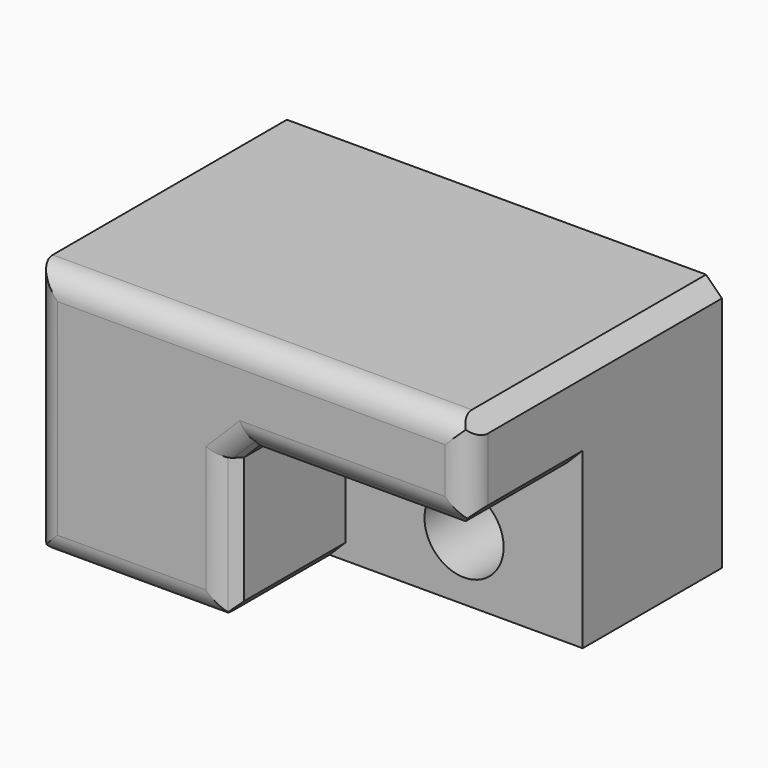
from build123d import *

# Parameters (mm, degrees)
F0_W         = 55
F0_H         = 32
F1_DEPTH     = 40
F2_W         = 30
F2_H         = 18
F3_DEPTH     = 20
F4_R         = 5
F5_DEPTH     = 22.001
F6_SIZE      = 2
F7_T1_DEPTH  = 36
F7_T3_DEPTH  = 45
F7_T5_DEPTH  = 68
F7_T7_DEPTH  = 23
F7_T12_DEPTH = 34.2132034356
F7_T17_DEPTH = 24.2132034356
F7_T22_DEPTH = 13.4214256026
F7_T29_DEPTH = 34.2132034356
F7_T33_DEPTH = 13.4214256026
F7_T40_DEPTH = 13.4214256026
F7_T44_DEPTH = 24.2132034356


# Not quite as in the source:
# - a fillet or chamfer that OpenCascade refuses, or shapes differently, is made with other operations: its cross-section is extruded or revolved along the edge and cut away or added


with BuildPart() as f1:
    # F0 (on Front) → F1 (new body)
    with BuildSketch(Plane.XZ):
        with Locations((27.5, -16)):
            Rectangle(F0_W, F0_H)
    extrude(amount=F1_DEPTH)

    # F2 (on face) → F3 (cut)
    with BuildSketch(Plane(origin=(0, 0, -32), x_dir=(1, 0, 0), z_dir=(0, 0, -1))):
        with Locations((40, 31)):
            Rectangle(F2_W, F2_H)
    extrude(amount=-F3_DEPTH, mode=Mode.SUBTRACT)

    # F4 (on face) → F5 (cut, through all)
    with BuildSketch(Plane.XZ.offset(22)):
        with Locations((40, -24)):
            Circle(F4_R)
    extrude(amount=-F5_DEPTH, mode=Mode.SUBTRACT)

    # F6
    f6_edges = [f1.edges().sort_by_distance(p)[0] for p in [
        (25, -40, -22),
        (25, -31, -32),
        (25, -31, -12),
        (55, -31, -12),
        (40, -40, -12),
        (55, -20, 0),
        (0, -20, -32),
    ]]
    chamfer(f6_edges, length=F6_SIZE)

    # F7: fillet of radius 3 on 7 edges, made by hand

    # F7_s2 → F7_t1 (cut)
    with BuildSketch(Plane.YZ.offset(-5.5)):
        with BuildLine():
            ThreePointArc((-40, -29), (-39.1213203436, -31.1213203436), (-37, -32))
            Line((-37, -32), (-40, -32))
            Line((-40, -32), (-40, -29))
        make_face()
    extrude(amount=F7_T1_DEPTH, mode=Mode.SUBTRACT)

    # F7_s4 → F7_t3 (cut)
    with BuildSketch(Plane.XY.offset(-37.5)):
        with BuildLine():
            ThreePointArc((0, -37), (0.8786796564, -39.1213203436), (3, -40))
            Line((3, -40), (0, -40))
            Line((0, -40), (0, -37))
        make_face()
    extrude(amount=F7_T3_DEPTH, mode=Mode.SUBTRACT)

    # F7_s6 → F7_t5 (cut)
    with BuildSketch(Plane.YZ.offset(-7.5)):
        with BuildLine():
            ThreePointArc((-37, 0), (-39.1213203436, -0.8786796564), (-40, -3))
            Line((-40, -3), (-40, 0))
            Line((-40, 0), (-37, 0))
        make_face()
    extrude(amount=F7_T5_DEPTH, mode=Mode.SUBTRACT)

    # F7_s8 → F7_t7 (cut)
    with BuildSketch(Plane.XY.offset(-17.5)):
        with BuildLine():
            ThreePointArc((52, -40), (54.1213203436, -39.1213203436), (55, -37))
            Line((55, -37), (55, -40))
            Line((55, -40), (52, -40))
        make_face()
    extrude(amount=F7_T7_DEPTH, mode=Mode.SUBTRACT)


with BuildPart() as f7_tool10:
    # F7_s11 → F7_t12 (new body)
    with BuildSketch(Plane.YZ.offset(58.1066017178)):
        with BuildLine():
            ThreePointArc((-40, -8.7573593129), (-39.7716385975, -9.90540961), (-39.1213203436, -10.8786796564))
            Line((-39.1213203436, -10.8786796564), (-40, -10))
            Line((-40, -10), (-40, -8.7573593129))
        make_face()
    extrude(amount=-F7_T12_DEPTH)

    split(bisect_by=Plane(origin=(25.6666666667, -25.6666666667, -25.6666666667), x_dir=(0.7071067812, 0.7071067812, 0), z_dir=(0.5773502692, -0.5773502692, -0.5773502692)), keep=Keep.TOP)


with BuildPart() as f1_1:
    add(f1.part)

    # F7_t9: cut F7_tool10
    add(f7_tool10.part, mode=Mode.SUBTRACT)


with BuildPart() as f7_tool15:
    # F7_s16 → F7_t17 (new body)
    with BuildSketch(Plane.XY.offset(-35.1066017178)):
        with BuildLine():
            ThreePointArc((21.7573593129, -40), (22.90540961, -39.7716385975), (23.8786796564, -39.1213203436))
            Line((23.8786796564, -39.1213203436), (23, -40))
            Line((23, -40), (21.7573593129, -40))
        make_face()
    extrude(amount=F7_T17_DEPTH)

    split(bisect_by=Plane(origin=(25.6666666667, -25.6666666667, -25.6666666667), x_dir=(0.7071067812, 0.7071067812, 0), z_dir=(0.5773502692, -0.5773502692, -0.5773502692)), keep=Keep.TOP)


with BuildPart() as f1_2:
    add(f1_1.part)

    # F7_t14: cut F7_tool15
    add(f7_tool15.part, mode=Mode.SUBTRACT)


with BuildPart() as f7_tool20:
    # F7_s21 → F7_t22 (new body)
    with BuildSketch(Plane(origin=(11.2451905284, 0, 11.2451905284), x_dir=(0, 1, 0), z_dir=(-0.7071067812, 0, -0.7071067812))):
        with BuildLine():
            ThreePointArc((-40, 24.6100366333), (-39.6642215019, 25.9891391634), (-38.7320508076, 27.0595263761))
            Line((-38.7320508076, 27.0595263761), (-40, 26.1629509039))
            Line((-40, 26.1629509039), (-40, 24.6100366333))
        make_face()
    extrude(amount=F7_T22_DEPTH)

    split(bisect_by=Plane(origin=(0, -25, -25), x_dir=(1, 0, 0), z_dir=(0, -0.7071067812, -0.7071067812)), keep=Keep.TOP)

    split(bisect_by=Plane(origin=(31.5, -31.5, 0), x_dir=(0, 0, 1), z_dir=(0.7071067812, -0.7071067812, 0)), keep=Keep.TOP)


with BuildPart() as f1_3:
    add(f1_2.part)

    # F7_t19: cut F7_tool20
    add(f7_tool20.part, mode=Mode.SUBTRACT)


with BuildPart() as f7_tool27:
    # F7_s28 → F7_t29 (new body)
    with BuildSketch(Plane.YZ.offset(58.1066017178)):
        with BuildLine():
            ThreePointArc((-40, -8.7573593129), (-39.7716385975, -9.90540961), (-39.1213203436, -10.8786796564))
            Line((-39.1213203436, -10.8786796564), (-40, -10))
            Line((-40, -10), (-40, -8.7573593129))
        make_face()
    extrude(amount=-F7_T29_DEPTH)

    split(bisect_by=Plane(origin=(25.6666666667, -25.6666666667, -25.6666666667), x_dir=(-0.7071067812, -0.7071067812, 0), z_dir=(-0.5773502692, 0.5773502692, 0.5773502692)), keep=Keep.TOP)


with BuildPart() as f7_tool31:
    # F7_s32 → F7_t33 (new body)
    with BuildSketch(Plane(origin=(11.2451905284, 0, 11.2451905284), x_dir=(0, 1, 0), z_dir=(-0.7071067812, 0, -0.7071067812))):
        with BuildLine():
            ThreePointArc((-40, 24.6100366333), (-39.6642215019, 25.9891391634), (-38.7320508076, 27.0595263761))
            Line((-38.7320508076, 27.0595263761), (-40, 26.1629509039))
            Line((-40, 26.1629509039), (-40, 24.6100366333))
        make_face()
    extrude(amount=F7_T33_DEPTH)

    split(bisect_by=Plane(origin=(0, -25, -25), x_dir=(1, 0, 0), z_dir=(0, 0.7071067812, 0.7071067812)), keep=Keep.TOP)


with BuildPart() as f7_tool27_1:
    add(f7_tool27.part)

    # F7_t35: intersect F7_tool31
    add(f7_tool31.part, mode=Mode.INTERSECT)


with BuildPart() as f1_4:
    add(f1_3.part)

    # F7_t25: cut F7_tool27
    add(f7_tool27_1.part, mode=Mode.SUBTRACT)


with BuildPart() as f7_tool38:
    # F7_s39 → F7_t40 (new body)
    with BuildSketch(Plane(origin=(11.2451905284, 0, 11.2451905284), x_dir=(0, 1, 0), z_dir=(-0.7071067812, 0, -0.7071067812))):
        with BuildLine():
            ThreePointArc((-40, 24.6100366333), (-39.6642215019, 25.9891391634), (-38.7320508076, 27.0595263761))
            Line((-38.7320508076, 27.0595263761), (-40, 26.1629509039))
            Line((-40, 26.1629509039), (-40, 24.6100366333))
        make_face()
    extrude(amount=F7_T40_DEPTH)

    split(bisect_by=Plane(origin=(31.5, -31.5, 0), x_dir=(0, 0, 1), z_dir=(-0.7071067812, 0.7071067812, 0)), keep=Keep.TOP)


with BuildPart() as f7_tool42:
    # F7_s43 → F7_t44 (new body)
    with BuildSketch(Plane.XY.offset(-35.1066017178)):
        with BuildLine():
            ThreePointArc((21.7573593129, -40), (22.90540961, -39.7716385975), (23.8786796564, -39.1213203436))
            Line((23.8786796564, -39.1213203436), (23, -40))
            Line((23, -40), (21.7573593129, -40))
        make_face()
    extrude(amount=F7_T44_DEPTH)

    split(bisect_by=Plane(origin=(25.6666666667, -25.6666666667, -25.6666666667), x_dir=(-0.7071067812, -0.7071067812, 0), z_dir=(-0.5773502692, 0.5773502692, 0.5773502692)), keep=Keep.TOP)


with BuildPart() as f7_tool38_1:
    add(f7_tool38.part)

    # F7_t46: intersect F7_tool42
    add(f7_tool42.part, mode=Mode.INTERSECT)


with BuildPart() as f1_5:
    add(f1_4.part)

    # F7_t36: cut F7_tool38
    add(f7_tool38_1.part, mode=Mode.SUBTRACT)


solid = f1_5.part
